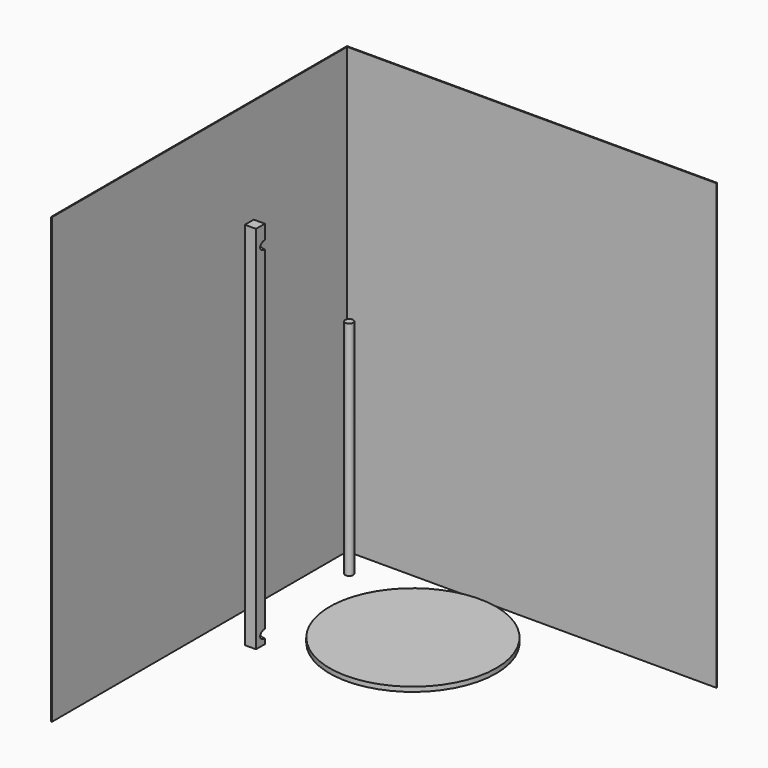
from build123d import *

# Parameters (mm, degrees)
F2_W      = 60
F2_H      = 60
F3_DEPTH  = 2000
F1_E1_W   = 2000
F1_E1_H   = 2400
F4_DEPTH  = 5
F1_E0_W   = 2000
F1_E0_H   = 2400
F5_DEPTH  = 5
F6_R      = 21.5
F7_DEPTH  = 1200
F10_DEPTH = 76
F12_R     = 450
F13_DEPTH = 25
F14_W     = 60
F14_H     = 60
F15_DEPTH = 400


# Not quite as in the source:
# - a pattern or mirror of a feature is missing from the dataset's text; its kind, count and spacing are read off the source's solid


with BuildPart() as f3:
    # F2 (on Top) → F3 (new body)
    with BuildSketch(Plane.XY):
        with Locations((233.3355557919, -913.7484741211)):
            Rectangle(F2_W, F2_H)
    extrude(amount=F3_DEPTH)

    # F9 (on face) → F10 (cut)
    with BuildSketch(Plane(origin=(-340.2064591646, -340.2064591646, 0), x_dir=(0.7071067812, -0.7071067812, 0), z_dir=(-0.7071067812, -0.7071067812, 0))):
        with BuildLine():
            ThreePointArc((833.6108961422, 1900), (827.0207987189, 1915.9099025767), (811.1108961422, 1922.5))
            Line((811.1108961422, 1922.5), (811.1108961422, 1877.5))
            ThreePointArc((811.1108961422, 1877.5), (827.0207987189, 1884.0900974233), (833.6108961422, 1900))
        make_face()
        with BuildLine():
            Line((811.1108961422, 1877.5), (811.1108961422, 1922.5))
            ThreePointArc((811.1108961422, 1922.5), (788.6108961422, 1900), (811.1108961422, 1877.5))
        make_face()
    f10 = extrude(amount=-F10_DEPTH, mode=Mode.SUBTRACT)

    # F10_copies: F10 across plane
    add(f10.mirror(Plane(origin=(0, 0, 975), x_dir=(-1, 0, 0), z_dir=(0, 0, -1))), mode=Mode.SUBTRACT)


with BuildPart() as f4:
    # F1_E1 (on explicit) → F4 (new body)
    with BuildSketch(Plane(origin=(0, 0, 0), x_dir=(0, -1, 0), z_dir=(-1, 0, 0))):
        with Locations((1000, 1200)):
            Rectangle(F1_E1_W, F1_E1_H)
    extrude(amount=-F4_DEPTH)

    # F1_E0 (on explicit) → F5 (join)
    with BuildSketch(Plane(origin=(2000, 0, 0), x_dir=(-1, 0, 0), z_dir=(0, 1, 0))):
        with Locations((1000, 1200)):
            Rectangle(F1_E0_W, F1_E0_H)
    extrude(amount=-F5_DEPTH)


with BuildPart() as f7:
    # F6 (on Top) → F7 (new body)
    with BuildSketch(Plane.XY):
        with Locations((138.325303793, -157.9697430134)):
            Circle(F6_R)
    extrude(amount=F7_DEPTH)


with BuildPart() as f13:
    # F12 (on Top) → F13 (new body)
    with BuildSketch(Plane.XY):
        with Locations((742.5876259804, -482.996404171)):
            Circle(F12_R)
    extrude(amount=F13_DEPTH)


with BuildPart() as f15:
    # F14 (on Front) → F15 (new body)
    with BuildSketch(Plane.XZ):
        with Locations((-205.0545227528, 30)):
            Rectangle(F14_W, F14_H)
    extrude(amount=F15_DEPTH)


solid = Compound([f3.part, f4.part, f7.part, f13.part, f15.part])
